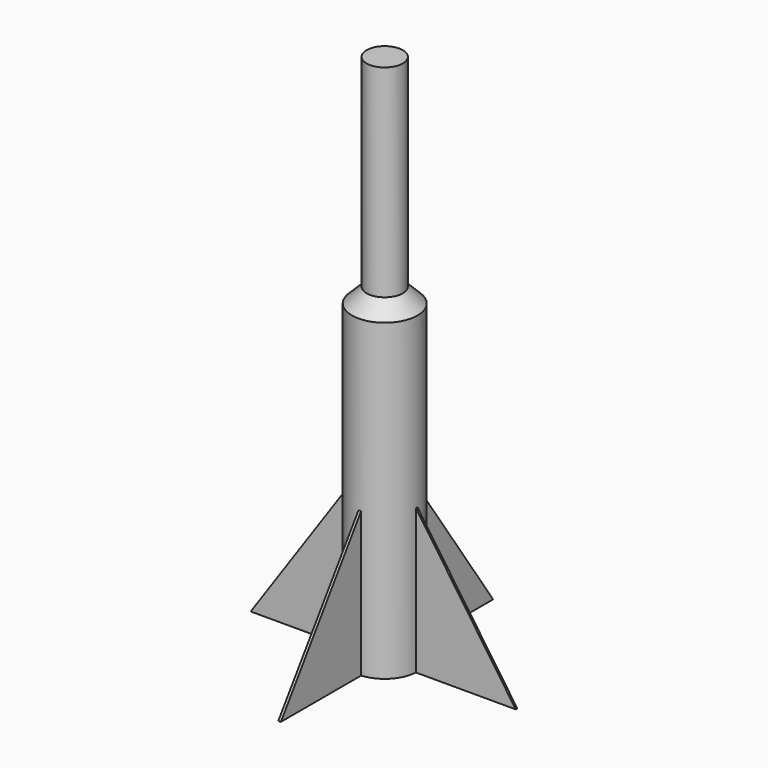
from build123d import *

# Parameters (mm, degrees)
F0_R        = 4.318
F1_DEPTH    = 44.45
F2_R        = 2.38125
F3_DEPTH    = 25.4
F4_S5_R     = 2.38125
F4_T6_DEPTH = 8
F5_W        = 0.3382458817
F5_H        = 13.1992071904
F6_DEPTH    = 19.05
F5_W_2      = 13.1341543086
F5_H_2      = 0.257695443
F5_H_3      = 13.1008949168
F5_W_3      = 13.120493669
F8_DEPTH    = 25.4
F10_DEPTH   = 25.4
F12_DEPTH   = 25.4
F14_DEPTH   = 25.4


# Not quite as in the source:
# - a fillet or chamfer that OpenCascade refuses, or shapes differently, is made with other operations: its cross-section is extruded or revolved along the edge and cut away or added


with BuildPart() as f1:
    # F0 (on Top) → F1 (new body)
    with BuildSketch(Plane.XY):
        Circle(F0_R)
    extrude(amount=F1_DEPTH)

    # F2 (on face) → F3 (join)
    with BuildSketch(Plane.XY.offset(44.45)):
        Circle(F2_R)
    extrude(amount=F3_DEPTH)

    # F4: chamfer of 3.175 on 1 edges, made by hand


with BuildPart() as f4_tool2:
    # F4_s3 → F4_t4 (revolve)
    with BuildSketch(Plane.XZ):
        Polygon((4.318, 41.275), (1.143, 44.45), (4.318, 44.45), align=None)
    revolve(axis=Axis((0, 0, 44.45), (0, 0, 1)))

    # F4_s5 → F4_t6 (cut, symmetric)
    with BuildSketch(Plane.XY.offset(42.9)):
        Circle(F4_S5_R)
    extrude(amount=F4_T6_DEPTH, both=True, mode=Mode.SUBTRACT)


with BuildPart() as f1_1:
    add(f1.part)

    # F4_t1: cut F4_tool2
    add(f4_tool2.part, mode=Mode.SUBTRACT)


with BuildPart() as f6:
    # F5 (on face) → F6 (new body)
    with BuildSketch(Plane(origin=(0, 0, 0), x_dir=(1, 0, 0), z_dir=(0, 0, -1))):
        with Locations((0.1691229409, 10.9176035952)):
            Rectangle(F5_W, F5_H)
    extrude(amount=-F6_DEPTH)

    # F7 (on face) → F8 (cut)
    with BuildSketch(Plane.YZ.offset(0.3382458817)):
        Polygon((-17.5172071904, 0), (-4.318, 19.05), (-17.5172071904, 19.05), align=None)
    extrude(amount=-F8_DEPTH, mode=Mode.SUBTRACT)


with BuildPart() as f6b:
    # F5 (on face) → F6, piece 2 (new body)
    with BuildSketch(Plane(origin=(0, 0, 0), x_dir=(1, 0, 0), z_dir=(0, 0, -1))):
        with Locations((10.8850771543, 0.1288477215)):
            Rectangle(F5_W_2, F5_H_2)
    extrude(amount=-F6_DEPTH)

    # F11 (on face) → F12 (cut)
    with BuildSketch(Plane.XZ.offset(0.257695443)):
        Polygon((17.4521543086, 19.05), (4.318, 19.05), (17.4521543086, 0), align=None)
    extrude(amount=-F12_DEPTH, mode=Mode.SUBTRACT)


with BuildPart() as f6c:
    # F5 (on face) → F6, piece 3 (new body)
    with BuildSketch(Plane(origin=(0, 0, 0), x_dir=(1, 0, 0), z_dir=(0, 0, -1))):
        with Locations((0.1691229409, -10.8684474584)):
            Rectangle(F5_W, F5_H_3)
    extrude(amount=-F6_DEPTH)

    # F9 (on face) → F10 (cut)
    with BuildSketch(Plane.YZ.offset(0.3382458817)):
        Polygon((17.4188949168, 19.05), (4.318, 19.05), (17.4188949168, 0), align=None)
    extrude(amount=-F10_DEPTH, mode=Mode.SUBTRACT)


with BuildPart() as f6d:
    # F5 (on face) → F6, piece 4 (new body)
    with BuildSketch(Plane(origin=(0, 0, 0), x_dir=(1, 0, 0), z_dir=(0, 0, -1))):
        with Locations((-10.8782468345, 0.1288477215)):
            Rectangle(F5_W_3, F5_H_2)
    extrude(amount=-F6_DEPTH)

    # F13 (on face) → F14 (cut)
    with BuildSketch(Plane.XZ.offset(0.257695443)):
        Polygon((-17.438493669, 0), (-4.318, 19.05), (-17.438493669, 19.05), align=None)
    extrude(amount=-F14_DEPTH, mode=Mode.SUBTRACT)


solid = Compound([f1_1.part, f6.part, f6b.part, f6c.part, f6d.part])
